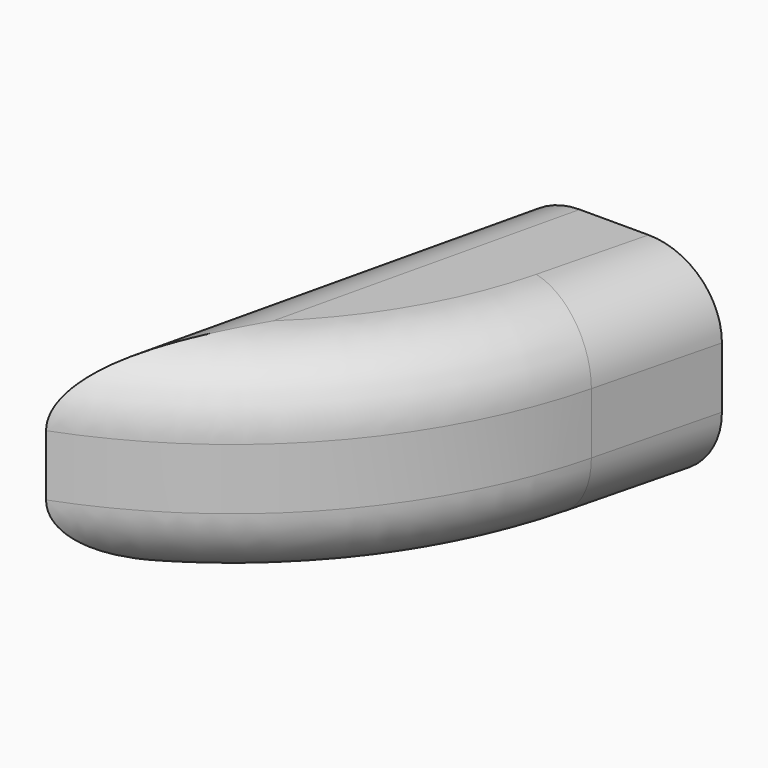
from build123d import *

# Parameters (mm, degrees)
F1_DEPTH = 50.8
F2_R     = 17.78
F3_R     = 17.78


# Not quite as in the source:
# - a feature names something its author has since deleted; it is built from what else it names


with BuildPart() as f1:
    # F0 (on Top) → F1 (new body)
    with BuildSketch(Plane.XY):
        with BuildLine():
            Line((3.2321710605, 7.2439061478), (-50.5689829588, 7.2439061478))
            Line((-50.5689829588, 7.2439061478), (-76.5684420406, -104.0992669462))
            ThreePointArc((-76.5684420406, -104.0992669462), (-30.6491711683, -72.8314970086), (-4.5715821907, -23.7783398479))
            Line((-4.5715821907, -23.7783398479), (3.2321710605, 7.2439061478))
        make_face()
    extrude(amount=F1_DEPTH)

    # F2
    f2_edges = [f1.edges().sort_by_distance(p)[0] for p in [
        (-0.669706, -8.267217, 50.8),
        (-63.568712, -48.42768, 50.8),
    ]]
    fillet(f2_edges, radius=F2_R)

    # F3
    f3_edges = [f1.edges().sort_by_distance(p)[0] for p in [
        (-0.669706, -8.267217, 0),
        (-63.568712, -48.42768, 0),
    ]]
    fillet(f3_edges, radius=F3_R)


solid = f1.part
